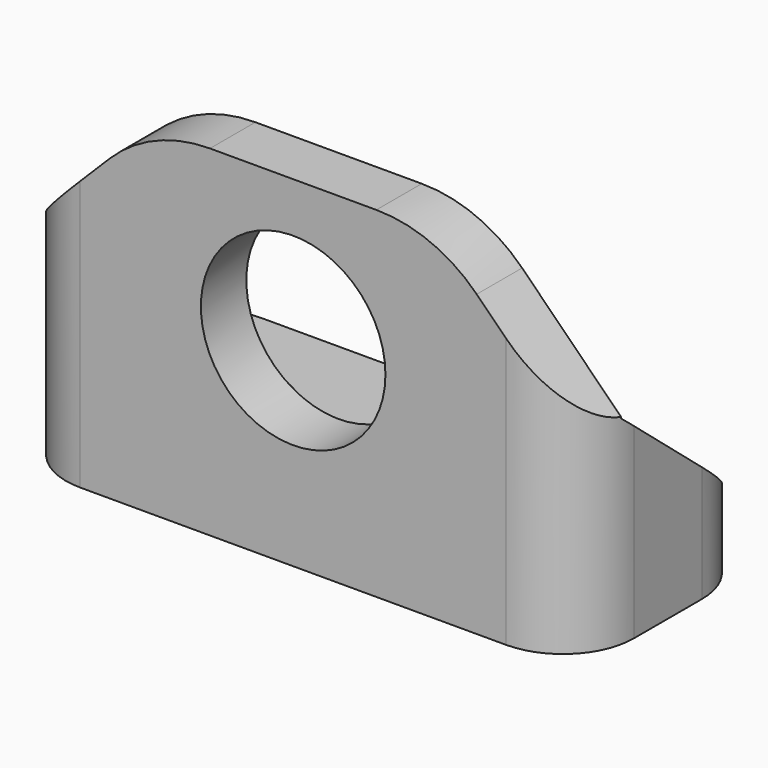
from build123d import *

# Parameters (mm, degrees)
F0_W         = 40
F0_H         = 16
F1_DEPTH     = 4
F2_W         = 40
F2_H         = 4
F3_DEPTH     = 20
F4_D         = 6
F12_D        = 13
F6_SIZE      = 10
F8_DEPTH     = 2
F9_DEPTH     = 2
F10_T1_DEPTH = 29
F10_T3_DEPTH = 39
F11_R        = 10


# Not quite as in the source:
# - a fillet or chamfer that OpenCascade refuses, or shapes differently, is made with other operations: its cross-section is extruded or revolved along the edge and cut away or added


with BuildPart() as f1:
    # F0 (on Top) → F1 (new body)
    with BuildSketch(Plane.XY):
        Rectangle(F0_W, F0_H)
    extrude(amount=F1_DEPTH)

    # F2 (on face) → F3 (join)
    with BuildSketch(Plane.XY.offset(4)):
        with Locations((0, -6)):
            Rectangle(F2_W, F2_H)
    extrude(amount=F3_DEPTH)

    # F4 (through all)
    with Locations(Plane.XY.offset(4)):
        with Locations((-10, 0), (10, 0)):
            Hole(F4_D / 2)

    # F12 (through all)
    with Locations(Plane(origin=(0, -4, 0), x_dir=(-1, 0, 0), z_dir=(0, 1, 0))):
        with Locations((0, 14)):
            Hole(F12_D / 2)

    # F6
    f6_edges = [f1.edges().sort_by_distance(p)[0] for p in [
        (-20, -6, 24),
        (20, -6, 24),
    ]]
    chamfer(f6_edges, length=F6_SIZE)

    # F7 (on face) → F8 (join)
    with BuildSketch(Plane(origin=(-20, 0, 0), x_dir=(0, -1, 0), z_dir=(-1, 0, 0))):
        Polygon((4, 14), (-8, 4), (4, 4), align=None)
    extrude(amount=-F8_DEPTH)

    # F13 (on face) → F9 (join)
    with BuildSketch(Plane.YZ.offset(20)):
        Polygon((-4, 4), (8, 4), (-4, 14), align=None)
    extrude(amount=-F9_DEPTH)

    # F10: fillet of radius 5 on 4 edges, made by hand

    # F10_s2 → F10_t1 (cut)
    with BuildSketch(Plane.XY.offset(-12.5)):
        with BuildLine():
            ThreePointArc((20, 3), (18.5355339059, 6.5355339059), (15, 8))
            Line((15, 8), (20, 8))
            Line((20, 8), (20, 3))
        make_face()
        with BuildLine():
            ThreePointArc((-20, 3), (-18.5355339059, 6.5355339059), (-15, 8))
            Line((-15, 8), (-20, 8))
            Line((-20, 8), (-20, 3))
        make_face()
    extrude(amount=F10_T1_DEPTH, mode=Mode.SUBTRACT)

    # F10_s4 → F10_t3 (cut)
    with BuildSketch(Plane.XY.offset(-12.5)):
        with BuildLine():
            ThreePointArc((-15, -8), (-18.5355339059, -6.5355339059), (-20, -3))
            Line((-20, -3), (-20, -8))
            Line((-20, -8), (-15, -8))
        make_face()
        with BuildLine():
            ThreePointArc((15, -8), (18.5355339059, -6.5355339059), (20, -3))
            Line((20, -3), (20, -8))
            Line((20, -8), (15, -8))
        make_face()
    extrude(amount=F10_T3_DEPTH, mode=Mode.SUBTRACT)

    # F11
    f11_edges = [f1.edges().sort_by_distance(p)[0] for p in [
        (10, -6, 24),
        (-10, -6, 24),
    ]]
    fillet(f11_edges, radius=F11_R)


solid = f1.part
